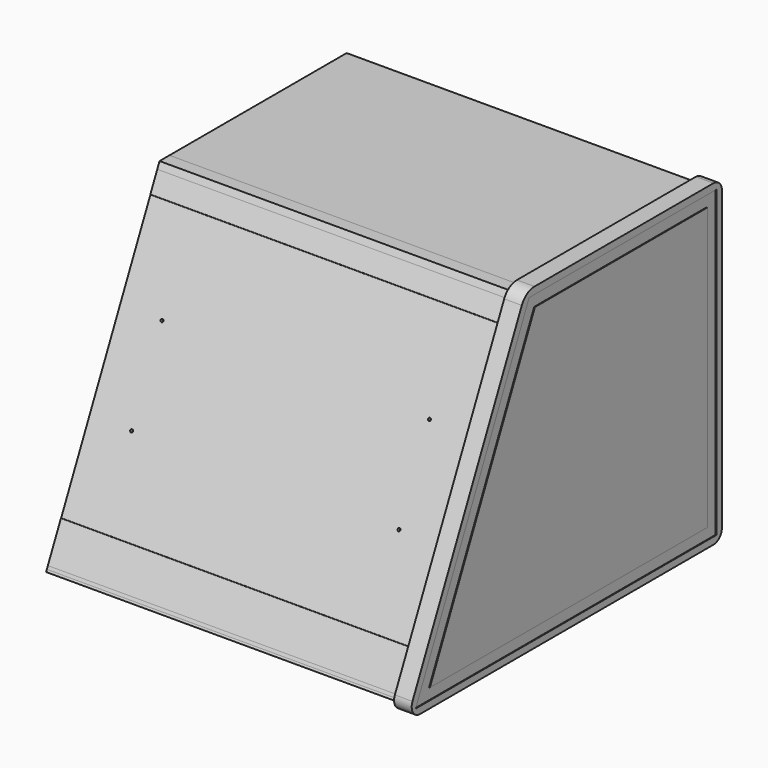
from build123d import *

# Parameters (mm, degrees)
F0_W      = 500
F0_H      = 500
F1_DEPTH  = 16
F3_W      = 500
F3_H      = 416
F4_DEPTH  = 16
F5_SIZE2  = 7.460913
F5_SIZE   = 15.99999
F7_DEPTH  = 500
F8_W      = 500
F8_H      = 500
F9_DEPTH  = 16
F11_DEPTH = 500
F13_DEPTH = 500.001
F15_DEPTH = 25
F16_R     = 15
F17_R     = 25
F18_R     = 15
F20_DEPTH = 1
F21_W     = 499.6
F21_H     = 375.1
F21_R     = 2
F22_DEPTH = 5
F24_DEPTH = 1


# Not quite as in the source:
# - a fillet or chamfer is up to 0.001 mm smaller than in the source, because OpenCascade refuses the exact size


with BuildPart() as f1:
    # F0 (on Top) → F1 (new body)
    with BuildSketch(Plane.XY):
        Rectangle(F0_W, F0_H)
    extrude(amount=F1_DEPTH)

    # F5 (size 16 and 7.4609225305 in the source; OpenCascade refuses exactly that, so slightly less here)
    f5_edges = [f1.edges().sort_by_distance(p)[0] for p in [
        (0, -250, 16),
    ]]
    f5_side = f1.faces().sort_by_distance((0, -250, 8))[0]
    chamfer(f5_edges, length=F5_SIZE, length2=F5_SIZE2, reference=f5_side)


with BuildPart() as f4:
    # F3 (on offset) → F4 (new body)
    with BuildSketch(Plane.XZ.offset(-250)):
        with Locations((0, 208)):
            Rectangle(F3_W, F3_H)
    extrude(amount=-F4_DEPTH)


with BuildPart() as f7:
    # F6 (on face) → F7 (new body, through all)
    with BuildSketch(Plane.YZ.offset(250)):
        Polygon((-264.5146755492, 0), (-250, 0), (-224.6429042956, 54.3784672222), (-234.612289953, 59.0272681013), (-236.7253812617, 54.4957291662), (-241.2569201968, 56.6088204749), (-264.5009245926, 6.7618921879), (-266.3272911232, 2.8452365235), (-267.6540467034, 0), align=None)
    extrude(amount=-F7_DEPTH)


with BuildPart() as f9:
    # F8 (on face) → F9 (new body)
    with BuildSketch(Plane.XY.offset(416)):
        with Locations((0, 16)):
            Rectangle(F8_W, F8_H)
    extrude(amount=F9_DEPTH)

    # F12 (on face) → F13 (cut, through all)
    with BuildSketch(Plane.YZ.offset(250)):
        Polygon((-78.702301391, 367.3491001344), (-31.9454936648, 467.6193978841), (-288.1607642735, 474.7963037545), (-288.1607642735, 367.3491001344), align=None)
    extrude(amount=-F13_DEPTH, mode=Mode.SUBTRACT)


with BuildPart() as f11:
    # F10 (on face) → F11 (new body, through all)
    with BuildSketch(Plane.YZ.offset(250)):
        Polygon((-70.1759296293, 385.6339633841), (-48.555091677, 432), (-56.6530844683, 432), (-66.2091383804, 432), (-70.2477012739, 423.3392739261), (-82.5637629132, 396.9273945071), (-78.032223978, 394.8143031984), (-80.1453152867, 390.2827642632), align=None)
    extrude(amount=-F11_DEPTH)


with BuildPart() as f15:
    # F14 (on face) → F15 (new body)
    with BuildSketch(Plane.YZ.offset(250)):
        Polygon((276, -10), (276, 442), (-72.5798409885, 442), (-283.3509024746, -10), align=None)
    extrude(amount=F15_DEPTH)

    # F16
    f16_edges = [f15.edges().sort_by_distance(p)[0] for p in [
        (262.5, 276, -10),
        (262.5, -283.350902, -10),
    ]]
    fillet(f16_edges, radius=F16_R)

    # F17
    f17_edges = [f15.edges().sort_by_distance(p)[0] for p in [
        (262.5, -72.579841, 442),
    ]]
    fillet(f17_edges, radius=F17_R)

    # F18
    f18_edges = [f15.edges().sort_by_distance(p)[0] for p in [
        (262.5, 276, 442),
    ]]
    fillet(f18_edges, radius=F18_R)

    # F19 (on face) → F20 (cut)
    with BuildSketch(Plane(origin=(250, 0, 0), x_dir=(0, -1, 0), z_dir=(-1, 0, 0))):
        Polygon((-266, 0), (267.6540467034, 0), (66.2091383804, 432), (-266, 432), align=None)
        Polygon((-250, 16), (-250, 416), (56.0160142075, 416), (242.5390774695, 16), align=None, mode=Mode.SUBTRACT)
    extrude(amount=-F20_DEPTH, mode=Mode.SUBTRACT)

    # F23 (on face) → F24 (cut)
    with BuildSketch(Plane.YZ.offset(275)):
        Polygon((266, 0), (266, 432), (-66.2091383804, 432), (-267.6540467034, 0), align=None)
        Polygon((-56.0160142075, 416), (250, 416), (250, 16), (-242.5390774695, 16), align=None, mode=Mode.SUBTRACT)
    extrude(amount=-F24_DEPTH, mode=Mode.SUBTRACT)


with BuildPart() as f22:
    # F21 (on face) → F22 (new body)
    with BuildSketch(Plane(origin=(0, -215.3178368682, 100.404356269), x_dir=(1, 0, 0), z_dir=(0, -0.906307787, 0.4226182617))):
        with Locations((0, 137.0954345648)):
            Rectangle(F21_W, F21_H)
        with Locations((-190, 68.6454345648)):
            Circle(F21_R, mode=Mode.SUBTRACT)
        with Locations((189.8, 68.6454345648)):
            Circle(F21_R, mode=Mode.SUBTRACT)
        with Locations((-190, 196.6454345648)):
            Circle(F21_R, mode=Mode.SUBTRACT)
        with Locations((189.8, 196.6454345648)):
            Circle(F21_R, mode=Mode.SUBTRACT)
    extrude(amount=F22_DEPTH)


solid = Compound([f1.part, f4.part, f7.part, f9.part, f11.part, f15.part, f22.part])
